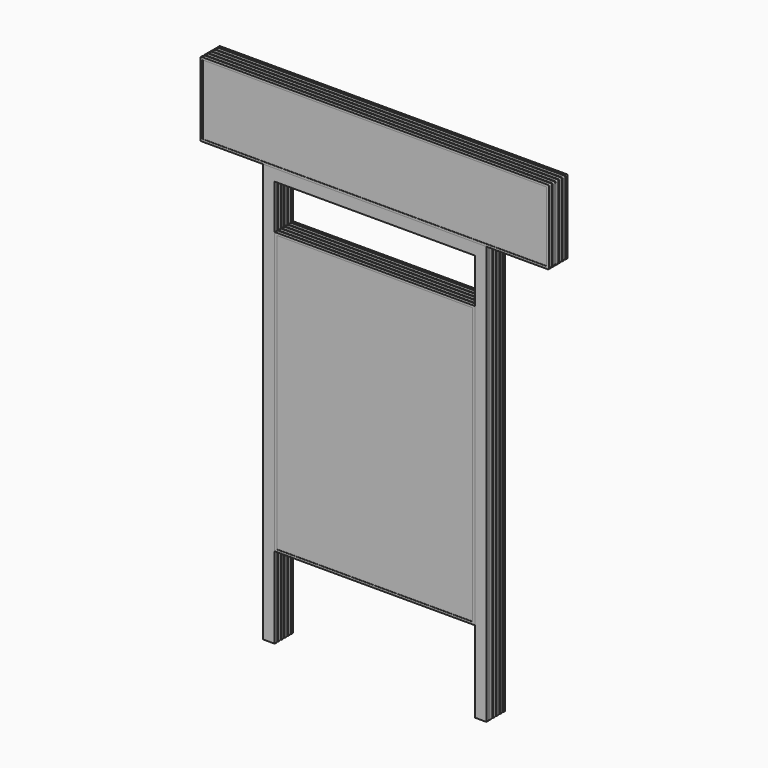
from build123d import *

# Parameters (mm, degrees)
F0_W      = 50
F0_H      = 1800
F1_DEPTH  = 100
F2_W      = 1500
F2_H      = 100
F3_DEPTH  = 320
F4_W      = 1480
F4_H      = 300
F5_DEPTH  = 100.001
F6_W      = 8
F6_H      = 2
F7_DEPTH  = 1500.001
F9_W      = 1480
F9_H      = 300
F10_DEPTH = 98
F11_W     = 2
F11_H     = 8
F12_DEPTH = 2120.001
F13_W     = 861
F13_H     = 50
F14_DEPTH = 100
F15_W     = 861
F15_H     = 1209
F15_W_2   = 841
F15_H_2   = 1189
F16_DEPTH = 100
F17_W     = 841
F17_H     = 1189
F18_DEPTH = 98
F19_W     = 8
F19_H     = 2
F20_DEPTH = 1180.501
F21_R     = 5
F22_W     = 2
F22_H     = 8
F23_DEPTH = 2120.001
F24_W     = 2
F24_H     = 8


# Not quite as in the source:
# - a feature of the source that left no trace in its solid (it failed there, or was rolled back) is left out


with BuildPart() as f1:
    # F0 (on Front) → F1 (new body)
    with BuildSketch(Plane.XZ):
        with Locations((-455.5, -900)):
            Rectangle(F0_W, F0_H)
    extrude(amount=F1_DEPTH)



with BuildPart() as f1b:
    # F0 (on Front) → F1, piece 2 (new body)
    with BuildSketch(Plane.XZ):
        with Locations((455.5, -900)):
            Rectangle(F0_W, F0_H)
    extrude(amount=F1_DEPTH)


with BuildPart() as f3:
    # F2 (on face) → F3 (new body)
    with BuildSketch(Plane.XY):
        with Locations((0, -50)):
            Rectangle(F2_W, F2_H)
    extrude(amount=F3_DEPTH)

    # F4 (on face) → F5 (cut, through all)
    with BuildSketch(Plane.XZ.offset(100)):
        with Locations((0, 160)):
            Rectangle(F4_W, F4_H)
    extrude(amount=-F5_DEPTH, mode=Mode.SUBTRACT)

    # F6 (on face) → F7 (cut, through all)
    with BuildSketch(Plane.YZ.offset(750)):
        with Locations((-86, 319)):
            Rectangle(F6_W, F6_H)
        with Locations((-68, 319)):
            Rectangle(F6_W, F6_H)
        with Locations((-50, 319)):
            Rectangle(F6_W, F6_H)
        with Locations((-32, 319)):
            Rectangle(F6_W, F6_H)
        with Locations((-14, 319)):
            Rectangle(F6_W, F6_H)
        with Locations((-14, 1)):
            Rectangle(F6_W, F6_H)
        with Locations((-32, 1)):
            Rectangle(F6_W, F6_H)
        with Locations((-86, 1)):
            Rectangle(F6_W, F6_H)
        with Locations((-68, 1)):
            Rectangle(F6_W, F6_H)
        with Locations((-50, 1)):
            Rectangle(F6_W, F6_H)
    extrude(amount=-F7_DEPTH, mode=Mode.SUBTRACT)

    # F11 (on face) → F12 (cut, through all)
    with BuildSketch(Plane.XY.offset(320)):
        with Locations((-749, -14)):
            Rectangle(F11_W, F11_H)
        with Locations((-749, -32)):
            Rectangle(F11_W, F11_H)
        with Locations((-749, -50)):
            Rectangle(F11_W, F11_H)
        with Locations((-749, -68)):
            Rectangle(F11_W, F11_H)
        with Locations((-749, -86)):
            Rectangle(F11_W, F11_H)
        with Locations((749, -50)):
            Rectangle(F11_W, F11_H)
        with Locations((749, -32)):
            Rectangle(F11_W, F11_H)
        with Locations((749, -68)):
            Rectangle(F11_W, F11_H)
        with Locations((749, -14)):
            Rectangle(F11_W, F11_H)
        with Locations((749, -86)):
            Rectangle(F11_W, F11_H)
    extrude(amount=-F12_DEPTH, mode=Mode.SUBTRACT)

    # F21
    f21_edges = [f3.edges().sort_by_distance(p)[0] for p in [
        (750, -95, 0),
        (748, -86, 2),
        (750, -77, 0),
        (748, -68, 2),
        (750, -59, 0),
        (748, -50, 2),
        (750, -41, 0),
        (748, -32, 2),
        (750, -23, 0),
        (748, -14, 2),
        (750, -5, 0),
        (750, -95, 320),
        (748, -86, 318),
        (750, -77, 320),
        (748, -68, 318),
        (750, -59, 320),
        (748, -50, 318),
        (750, -41, 320),
        (748, -32, 318),
        (750, -23, 320),
        (748, -14, 318),
        (750, -5, 320),
        (-750, -5, 320),
        (-748, -14, 318),
        (-750, -23, 320),
        (-748, -32, 318),
        (-750, -41, 320),
        (-748, -50, 318),
        (-750, -59, 320),
        (-748, -68, 318),
        (-750, -77, 320),
        (-748, -86, 318),
        (-750, -95, 320),
        (-750, -95, 0),
        (-748, -86, 2),
        (-750, -77, 0),
        (-748, -68, 2),
        (-750, -59, 0),
        (-748, -50, 2),
        (-750, -41, 0),
        (-748, -32, 2),
        (-750, -23, 0),
        (-748, -14, 2),
        (-750, -5, 0),
    ]]
    fillet(f21_edges, radius=F21_R)


with BuildPart() as f10:
    # F9 (on offset) → F10 (new body, through all)
    with BuildSketch(Plane.XZ.offset(99)):
        with Locations((0, 160)):
            Rectangle(F9_W, F9_H)
    extrude(amount=-F10_DEPTH)


with BuildPart() as f1_1:
    add(f1.part)

    add(f1b.part)  # F14 merges F1b
    # F13 (on face) → F14 (join, through all)
    with BuildSketch(Plane(origin=(0, 0, 0), x_dir=(-1, 0, 0), z_dir=(0, 1, 0))):
        with Locations((0, -25)):
            Rectangle(F13_W, F13_H)
    extrude(amount=-F14_DEPTH)

    # F22 (on face) → F23 (cut, through all)
    with BuildSketch(Plane(origin=(0, 0, -1800), x_dir=(1, 0, 0), z_dir=(0, 0, -1))):
        with Locations((-479.5, 14)):
            Rectangle(F22_W, F22_H)
        with Locations((-479.5, 32)):
            Rectangle(F22_W, F22_H)
        with Locations((-479.5, 50)):
            Rectangle(F22_W, F22_H)
        with Locations((-479.5, 68)):
            Rectangle(F22_W, F22_H)
        with Locations((-479.5, 86)):
            Rectangle(F22_W, F22_H)
        with Locations((479.5, 86)):
            Rectangle(F22_W, F22_H)
        with Locations((479.5, 14)):
            Rectangle(F22_W, F22_H)
        with Locations((479.5, 50)):
            Rectangle(F22_W, F22_H)
        with Locations((479.5, 68)):
            Rectangle(F22_W, F22_H)
        with Locations((479.5, 32)):
            Rectangle(F22_W, F22_H)
    extrude(amount=-F23_DEPTH, mode=Mode.SUBTRACT)

    # F25: sweep along a path in F25_path
    with BuildLine(Plane(origin=(-430.5, -100, -50), x_dir=(0, 0, -1), z_dir=(0, 1, 0))) as f25_path:
        Line((1750, 0), (0, 0))
        Line((0, 0), (0, -861))
        Line((0, -861), (1750, -861))
    # F24 (on face) → F25 (sweep, cut)
    with BuildSketch(Plane(origin=(0, 0, -1800), x_dir=(1, 0, 0), z_dir=(0, 0, -1))):
        with Locations((-431.5, 86)):
            Rectangle(F24_W, F24_H)
        with Locations((-431.5, 14)):
            Rectangle(F24_W, F24_H)
        with Locations((-431.5, 32)):
            Rectangle(F24_W, F24_H)
        with Locations((-431.5, 50)):
            Rectangle(F24_W, F24_H)
        with Locations((-431.5, 68)):
            Rectangle(F24_W, F24_H)
    sweep(path=f25_path.line, transition=Transition.RIGHT, mode=Mode.SUBTRACT)


with BuildPart() as f16:
    # F15 (on face) → F16 (new body)
    with BuildSketch(Plane.XZ.offset(100)):
        with Locations((0, -845.5)):
            Rectangle(F15_W, F15_H)
        with Locations((0, -845.5)):
            Rectangle(F15_W_2, F15_H_2, mode=Mode.SUBTRACT)
    extrude(amount=-F16_DEPTH)

    # F17 (on face) → F18 (join, through all)
    with BuildSketch(Plane.XZ.offset(99)):
        with Locations((0, -845.5)):
            Rectangle(F17_W, F17_H)
    extrude(amount=-F18_DEPTH)

    # F19 (on face) → F20 (cut, through all)
    with BuildSketch(Plane.YZ.offset(430.5)):
        with Locations((-86, -242)):
            Rectangle(F19_W, F19_H)
        with Locations((-68, -242)):
            Rectangle(F19_W, F19_H)
        with Locations((-50, -242)):
            Rectangle(F19_W, F19_H)
        with Locations((-32, -242)):
            Rectangle(F19_W, F19_H)
        with Locations((-14, -242)):
            Rectangle(F19_W, F19_H)
        with Locations((-86, -1449)):
            Rectangle(F19_W, F19_H)
        with Locations((-68, -1449)):
            Rectangle(F19_W, F19_H)
        with Locations((-50, -1449)):
            Rectangle(F19_W, F19_H)
        with Locations((-14, -1449)):
            Rectangle(F19_W, F19_H)
        with Locations((-32, -1449)):
            Rectangle(F19_W, F19_H)
    extrude(amount=-F20_DEPTH, mode=Mode.SUBTRACT)


solid = Compound([f3.part, f10.part, f1_1.part, f16.part])
